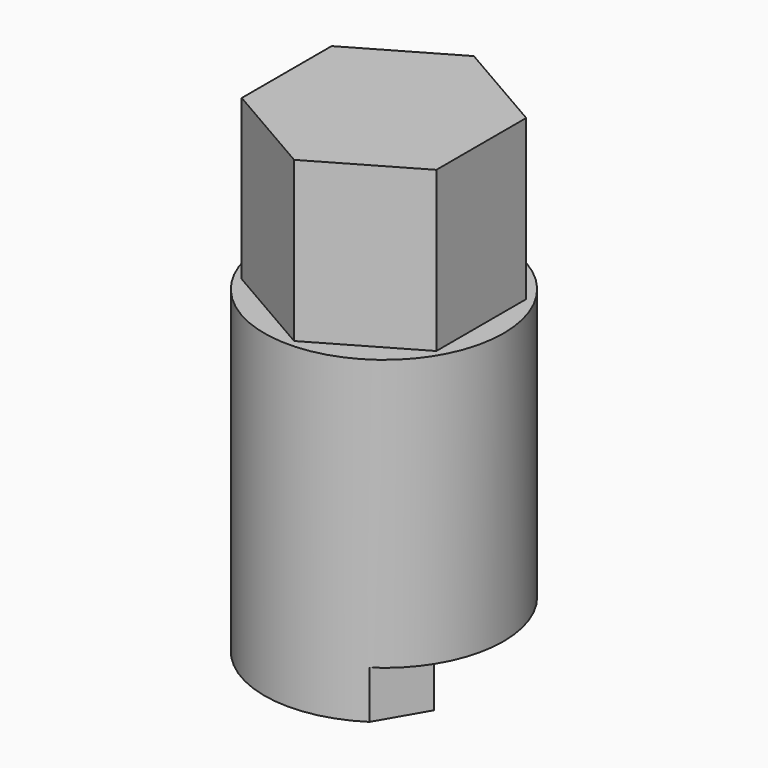
from build123d import *

# Parameters (mm, degrees)
F0_R      = 7.5
F1_DEPTH  = 30
F2_R      = 4.25
F3_DEPTH  = 20
F4_R      = 4.25
F5_DEPTH  = 3
F7_R      = 7.5
F8_DEPTH  = 10
F10_DEPTH = 3


# Not quite as in the source:
# - a feature names something its author has since deleted; it is built from what else it names


with BuildPart() as f1:
    # F0 (on Top) → F1 (new body)
    with BuildSketch(Plane.XY):
        Circle(F0_R)
    extrude(amount=F1_DEPTH)

    # F2 (on face) → F3 (cut)
    with BuildSketch(Plane(origin=(0, 0, 0), x_dir=(1, 0, 0), z_dir=(0, 0, -1))):
        Circle(F2_R)
    extrude(amount=-F3_DEPTH, mode=Mode.SUBTRACT)

    # F4 (on face) → F5 (cut)
    with BuildSketch(Plane(origin=(0, 0, 0), x_dir=(1, 0, 0), z_dir=(0, 0, -1))):
        Polygon((5.8, -3.3486315613), (5.8, 3.3486315613), (0, 6.6972631226), (-5.8, 3.3486315613), (-5.8, -3.3486315613), (0, -6.6972631226), align=None)
        Circle(F4_R, mode=Mode.SUBTRACT)
    extrude(amount=-F5_DEPTH, mode=Mode.SUBTRACT)

    # F7 (on face) → F8 (cut)
    with BuildSketch(Plane.XY.offset(30)):
        Circle(F7_R)
        Polygon((0, 7.0436732841), (6.1, 3.5218366421), (6.1, -3.5218366421), (0, -7.0436732841), (-6.1, -3.5218366421), (-6.1, 3.5218366421), align=None, mode=Mode.SUBTRACT)
    extrude(amount=-F8_DEPTH, mode=Mode.SUBTRACT)

    # F9 (on face) → F10 (cut, through all)
    with BuildSketch(Plane(origin=(0, 0, 0), x_dir=(1, 0, 0), z_dir=(0, 0, -1))):
        with BuildLine():
            Line((4.1120525285, 6.2722423425), (5.8, 3.3486315613))
            Line((5.8, 3.3486315613), (5.8, -3.3486315613))
            Line((5.8, -3.3486315613), (0, -6.6972631226))
            Line((0, -6.6972631226), (-3.3758949431, -6.6972631226))
            ThreePointArc((-3.3758949431, -6.6972631226), (3.9326065101, -6.3862826462), (7.5, 0))
            ThreePointArc((7.5, 0), (6.5988784639, 3.5643797523), (4.1120525285, 6.2722423425))
        make_face()
    extrude(amount=-F10_DEPTH, mode=Mode.SUBTRACT)


solid = f1.part
